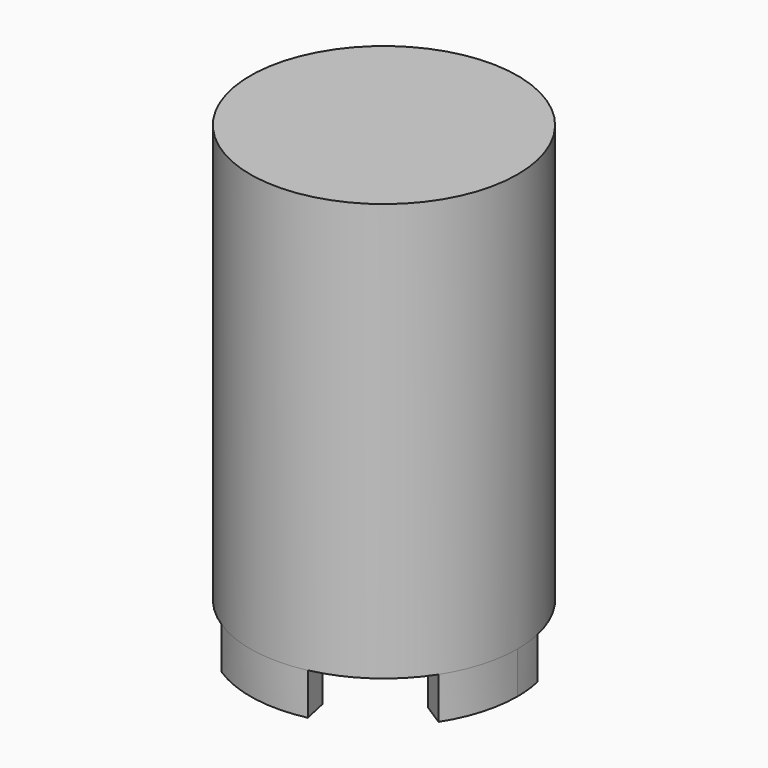
from build123d import *

# Parameters (mm, degrees)
F0_R     = 16
F1_DEPTH = 50
F3_DEPTH = 5


# Not quite as in the source:
# - after a boolean that leaves OpenCascade's solid faulty, fix() repairs it


with BuildPart() as f1:
    # F0 (on Top) → F1 (new body)
    with BuildSketch(Plane.XY):
        with Locations((41.4022505283, -34.313749522)):
            Circle(F0_R)
    extrude(amount=F1_DEPTH)

    # F2 (on face) → F3 (join)
    with BuildSketch(Plane(origin=(0, 0, 0), x_dir=(1, 0, 0), z_dir=(0, 0, -1))):
        Polygon((57.0387140238, 30.9224357125), (54.8569208916, 42.9723779016), (52.2755180634, 41.3111400427), (54.0387140238, 31.573090602), align=None)
        with BuildLine():
            ThreePointArc((57.0387140238, 30.9224357125), (57.3111068029, 32.6083779976), (57.4022505283, 34.313749522))
            ThreePointArc((57.4022505283, 34.313749522), (56.7527346544, 38.8262473994), (54.8569208916, 42.9723779016))
            Line((54.8569208916, 42.9723779016), (57.0387140238, 30.9224357125))
        make_face()
        Polygon((38.0109367189, 18.6772860265), (50.060878908, 20.8590791587), (48.399641049, 23.4404819869), (38.6615916084, 21.6772860265), align=None)
        with BuildLine():
            ThreePointArc((38.0109367189, 18.6772860265), (44.252900632, 18.5697413288), (50.060878908, 20.8590791587))
            Line((50.060878908, 20.8590791587), (38.0109367189, 18.6772860265))
        make_face()
        Polygon((28.7657870328, 37.0544084419), (25.7657870328, 37.7050633314), (27.9475801651, 25.6551211423), (30.5289829933, 27.3163590013), align=None)
        with BuildLine():
            Line((27.9475801651, 25.6551211423), (25.7657870328, 37.7050633314))
            ThreePointArc((25.7657870328, 37.7050633314), (25.6582423352, 31.4630994183), (27.9475801651, 25.6551211423))
        make_face()
        Polygon((44.1429094483, 46.9502130175), (44.7935643378, 49.9502130175), (32.7436221487, 47.7684198852), (34.4048600077, 45.187017057), align=None)
        with BuildLine():
            Line((32.7436221487, 47.7684198852), (44.7935643378, 49.9502130175))
            ThreePointArc((44.7935643378, 49.9502130175), (38.5516004247, 50.0577577151), (32.7436221487, 47.7684198852))
        make_face()
    extrude(amount=F3_DEPTH)

    add(f1.part.fix(), mode=Mode.REPLACE)


solid = f1.part
